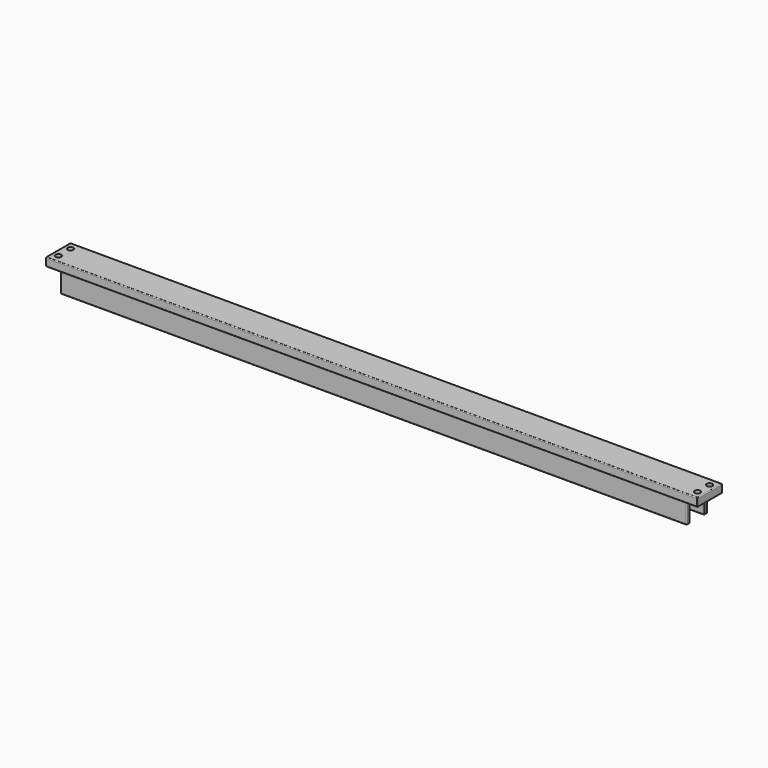
from build123d import *

# Parameters (mm, degrees)
F1_DEPTH = 390
F2_W     = 31
F2_H     = 25
F3_DEPTH = 15.5
F4_W     = 31
F4_H     = 25
F5_DEPTH = 15.5
F6_R     = 2
F7_DEPTH = 10.001
F8_R     = 3.5
F9_DEPTH = 4
F10_R    = 1
F11_R    = 1


# Not quite as in the source:
# - a pattern or mirror of a feature is missing from the dataset's text; its kind, count and spacing are read off the source's solid


with BuildPart() as f1:
    # F0 (on Right) → F1 (new body, symmetric)
    with BuildSketch(Plane.YZ):
        Polygon((18.5, 12.5), (-18.5, 12.5), (-18.5, 2.5), (-15.5, 2.5), (-15.5, -22.5), (-10.5, -22.5), (-10.5, 2.5), (0, 2.5), (10.5, 2.5), (10.5, -22.5), (15.5, -22.5), (15.5, 2.5), (18.5, 2.5), align=None)
    extrude(amount=F1_DEPTH, both=True)

    # F2 (on face) → F3 (cut)
    with BuildSketch(Plane(origin=(-390, 0, 0), x_dir=(0, -1, 0), z_dir=(-1, 0, 0))):
        with Locations((0, -10)):
            Rectangle(F2_W, F2_H)
    extrude(amount=-F3_DEPTH, mode=Mode.SUBTRACT)

    # F4 (on face) → F5 (cut)
    with BuildSketch(Plane.YZ.offset(390)):
        with Locations((0, -10)):
            Rectangle(F4_W, F4_H)
    extrude(amount=-F5_DEPTH, mode=Mode.SUBTRACT)

    # F6 (on face) → F7 (cut, through all)
    with BuildSketch(Plane(origin=(0, 0, 2.5), x_dir=(1, 0, 0), z_dir=(0, 0, -1))):
        with Locations((-382.25, 9)):
            Circle(F6_R)
        with Locations((-382.25, -9)):
            Circle(F6_R)
    f7 = extrude(amount=-F7_DEPTH, mode=Mode.SUBTRACT)

    # F7_copies: F7 across plane
    add(f7.mirror(Plane(origin=(0, 0, 0), x_dir=(0, 0, 1), z_dir=(1, 0, 0))), mode=Mode.SUBTRACT)

    # F8 (on face) → F9 (cut)
    with BuildSketch(Plane.XY.offset(12.5)):
        with Locations((-382.25, -9)):
            Circle(F8_R)
        with Locations((-382.25, 9)):
            Circle(F8_R)
    f9 = extrude(amount=-F9_DEPTH, mode=Mode.SUBTRACT)

    # F9_copies: F9 across plane
    add(f9.mirror(Plane(origin=(0, 0, 0), x_dir=(0, 0, 1), z_dir=(1, 0, 0))), mode=Mode.SUBTRACT)

    # F10
    f10_edges = [f1.edges().sort_by_distance(p)[0] for p in [
        (390, 18.5, 7.5),
        (390, -18.5, 7.5),
        (374.5, 13, -22.5),
        (374.5, -13, -22.5),
        (-390, -18.5, 7.5),
        (-374.5, -13, -22.5),
        (-374.5, 13, -22.5),
        (-390, 18.5, 7.5),
    ]]
    fillet(f10_edges, radius=F10_R)

    # F11
    f11_edges = [f1.edges().sort_by_distance(p)[0] for p in [
        (-374.5, -10.5, -9.5),
        (-374.5, -15.5, -9.5),
        (-374.5, 15.5, -9.5),
        (-374.5, 10.5, -9.5),
        (-374.5, 13, -21.5),
        (-374.5, 13, 2.5),
        (-390, 0, 2.5),
        (-390, 0, 12.5),
        (0, -15.5, 2.5),
        (-389.707107, 18.207107, 12.5),
        (-389.707107, -18.207107, 12.5),
        (0, 18.5, 12.5),
        (0, -18.5, 12.5),
        (389.707107, 18.207107, 12.5),
        (389.707107, -18.207107, 12.5),
        (390, 0, 12.5),
        (-389.707107, 18.207107, 2.5),
        (-389.707107, -18.207107, 2.5),
        (0, 18.5, 2.5),
        (0, -18.5, 2.5),
        (389.707107, 18.207107, 2.5),
        (389.707107, -18.207107, 2.5),
        (390, 0, 2.5),
        (-374.5, -13, 2.5),
        (374.5, -13, 2.5),
        (0, -10.5, 2.5),
        (0, 10.5, 2.5),
        (374.5, 13, 2.5),
        (0, 15.5, 2.5),
        (374.5, -15.5, -9.5),
        (374.207107, -15.5, -22.207107),
        (0, -15.5, -22.5),
        (-374.207107, -15.5, -22.207107),
        (374.5, -10.5, -9.5),
        (0, -10.5, -22.5),
        (-374.207107, -10.5, -22.207107),
        (374.207107, -10.5, -22.207107),
        (374.5, 10.5, -9.5),
        (374.207107, 10.5, -22.207107),
        (0, 10.5, -22.5),
        (-374.207107, 10.5, -22.207107),
        (374.5, 15.5, -9.5),
        (0, 15.5, -22.5),
        (-374.207107, 15.5, -22.207107),
        (374.207107, 15.5, -22.207107),
    ]]
    fillet(f11_edges, radius=F11_R)


solid = f1.part
